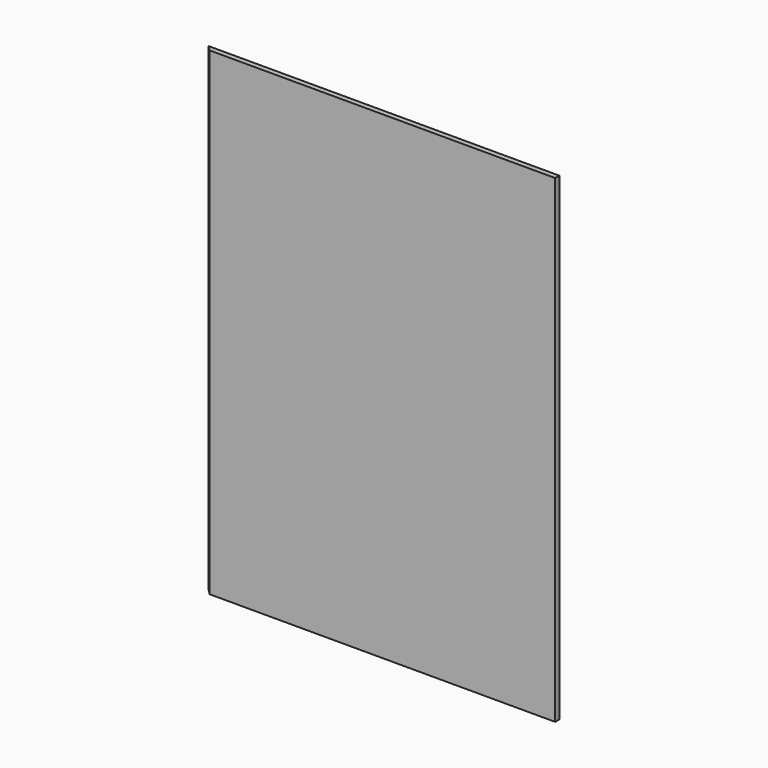
from build123d import *

# Parameters (mm, degrees)
F0_W        = 215.9
F0_H        = 292.1
F1_DEPTH    = 1.5875
F2_T1_DEPTH = 318.2282991577


# Not quite as in the source:
# - a fillet or chamfer that OpenCascade refuses, or shapes differently, is made with other operations: its cross-section is extruded or revolved along the edge and cut away or added


with BuildPart() as f1:
    # F0 (on Front) → F1 (new body, symmetric)
    with BuildSketch(Plane.XZ):
        Rectangle(F0_W, F0_H)
    extrude(amount=F1_DEPTH, both=True)

    # F2: chamfer of 5.08 on 1 edges, made by hand

    # F2_s2 → F2_t1 (cut)
    with BuildSketch(Plane.XY.offset(-159.1141495789)):
        Polygon((-102.87, -1.5875), (-107.95, 3.4925), (-107.95, -1.5875), align=None)
    extrude(amount=F2_T1_DEPTH, mode=Mode.SUBTRACT)


solid = f1.part
